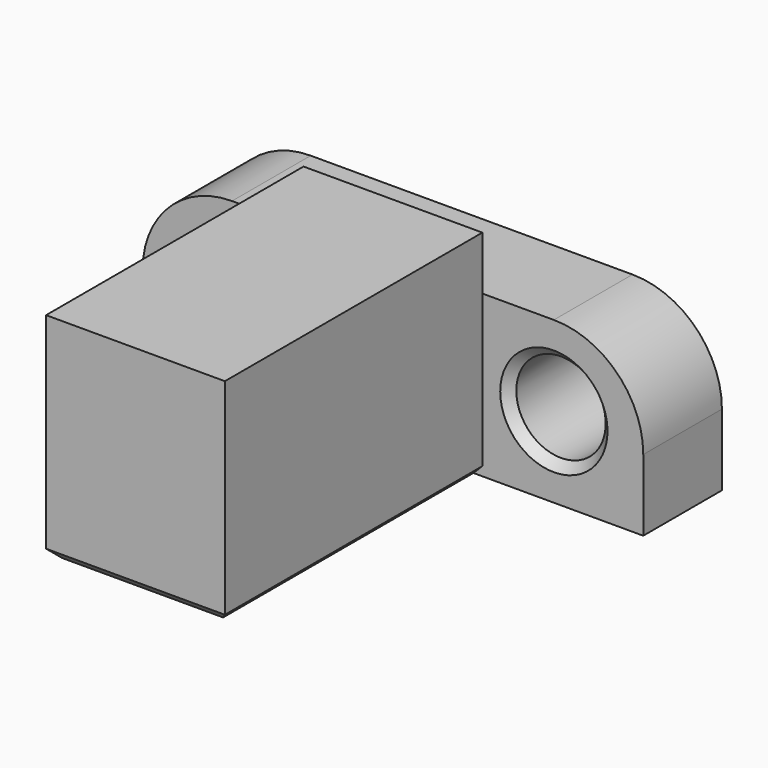
from build123d import *

# Parameters (mm, degrees)
F0_R     = 3
F1_DEPTH = 9
F3_D     = 5
F4_W     = 10
F4_H     = 18
F5_DEPTH = 3
F6_R     = 5
F7_SIZE  = 0.5


with BuildPart() as f1:
    # F0 (on Top) → F1 (new body)
    with BuildSketch(Plane.XY):
        Polygon((-5, -5.5), (5, -5.5), (5, 12.5), (14, 12.5), (14, 18), (-14, 18), (-14, 12.5), (-5, 12.5), align=None)
        Circle(F0_R, mode=Mode.SUBTRACT)
    extrude(amount=F1_DEPTH)

    # F3 (through all)
    with Locations(Plane.XZ.offset(-12.5)):
        with Locations((9, 4.5), (-9, 4.5)):
            Hole(F3_D / 2)

    # F4 (on face) → F5 (join)
    with BuildSketch(Plane.XY.offset(9)):
        with Locations((0, 3.5)):
            Rectangle(F4_W, F4_H)
    extrude(amount=F5_DEPTH)

    # F6
    f6_edges = [f1.edges().sort_by_distance(p)[0] for p in [
        (14, 15.25, 9),
        (-14, 15.25, 9),
    ]]
    fillet(f6_edges, radius=F6_R)

    # F7
    f7_edges = [f1.edges().sort_by_distance(p)[0] for p in [
        (-3, 0, 0),
        (5, 3.5, 0),
        (-5, 3.5, 0),
        (0, -5.5, 0),
        (-11.5, 12.5, 4.5),
        (6.5, 12.5, 4.5),
    ]]
    chamfer(f7_edges, length=F7_SIZE)


solid = f1.part
